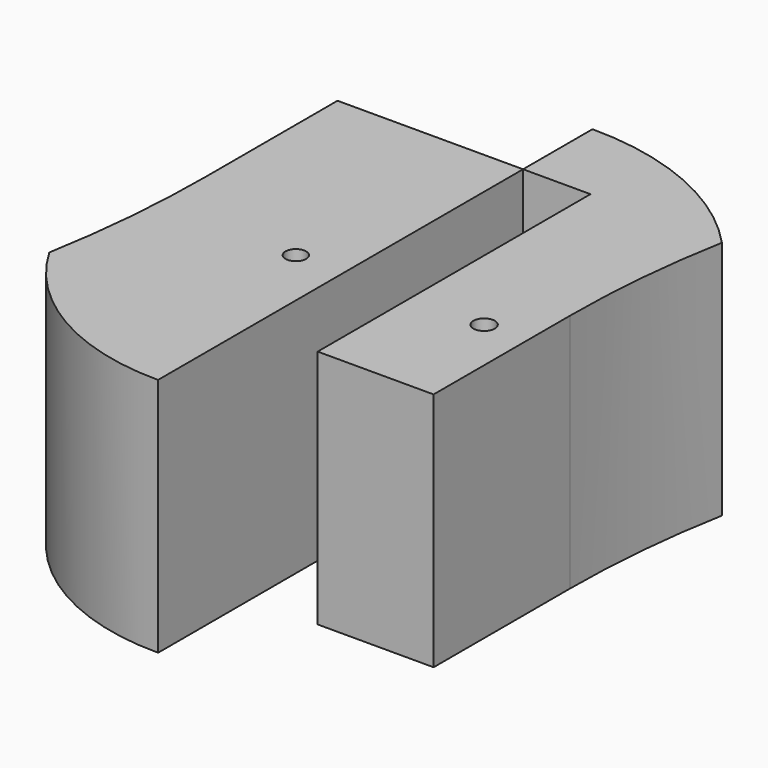
from build123d import *

# Parameters (mm, degrees)
F0_W     = 8.3915624609
F0_H     = 22
F0_R     = 0.6628669698
F0_W_2   = 0.0715297889
F0_H_2   = 12.9456651346
F1_DEPTH = 15.5
F0_W_3   = 5.9789330999
F0_R_2   = 0.68921597


with BuildPart() as f1:
    # F0 (on Top) → F1 (new body)
    with BuildSketch(Plane.XY):
        Polygon((-26.8058474948, -33.4269645675), (-29.3058474948, -33.4269645675), (-29.3058474948, -44.0262116721), (-29.3058474948, -55.4269645675), (-26.8058474948, -55.4269645675), align=None)
        with Locations((-22.6100662644, -44.4269645675)):
            Rectangle(F0_W, F0_H)
        with Locations((-20.4199831933, -47.8965379298)):
            Circle(F0_R, mode=Mode.SUBTRACT)
        with BuildLine():
            Line((-29.3058474948, -55.4269645675), (-29.3058474948, -44.0262116721))
            ThreePointArc((-29.3058474948, -44.0262116721), (-29.5554500968, -49.7483224557), (-30.3023617679, -55.4269645675))
            ThreePointArc((-30.3023617679, -55.4269645675), (-24.8175859802, -60.8874080585), (-17.334317706, -62.8622256441))
            Line((-17.334317706, -62.8622256441), (-17.334317706, -55.4269645675))
            Line((-17.334317706, -55.4269645675), (-18.4142850339, -55.4269645675))
            Line((-18.4142850339, -55.4269645675), (-26.8058474948, -55.4269645675))
            Line((-26.8058474948, -55.4269645675), (-29.3058474948, -55.4269645675))
        make_face()
        Polygon((-17.4058474948, -33.4269645675), (-18.4142850339, -33.4269645675), (-18.4142850339, -55.4269645675), (-17.334317706, -55.4269645675), (-17.334317706, -46.3726297021), (-17.4058474948, -46.3726297021), align=None)
        with Locations((-17.3700826004, -39.8997971348)):
            Rectangle(F0_W_2, F0_H_2)
    extrude(amount=F1_DEPTH)


with BuildPart() as f1b:
    # F0 (on Top) → F1, piece 2 (new body)
    with BuildSketch(Plane.XY):
        with BuildLine():
            ThreePointArc((-4.5023617679, -33.4269645675), (-10.3335838979, -29.2865306602), (-17.334317706, -27.8250004287))
            Line((-17.334317706, -27.8250004287), (-17.334317706, -33.4269645675))
            Line((-17.334317706, -33.4269645675), (-12.9847805947, -33.4269645675))
            Line((-12.9847805947, -33.4269645675), (-7.0058474948, -33.4269645675))
            Line((-7.0058474948, -33.4269645675), (-5.5058474948, -33.4269645675))
            Line((-5.5058474948, -33.4269645675), (-5.5058474948, -44.4269645675))
            ThreePointArc((-5.5058474948, -44.4269645675), (-5.2544562745, -38.9041259948), (-4.5023617679, -33.4269645675))
        make_face()
        with Locations((-9.9953140448, -44.4269645675)):
            Rectangle(F0_W_3, F0_H)
        with Locations((-8.2693165168, -47.8965379298)):
            Circle(F0_R_2, mode=Mode.SUBTRACT)
        Polygon((-5.5058474948, -55.4269645675), (-5.5058474948, -44.4269645675), (-5.5058474948, -33.4269645675), (-7.0058474948, -33.4269645675), (-7.0058474948, -55.4269645675), align=None)
    extrude(amount=F1_DEPTH)


solid = Compound([f1.part, f1b.part])
